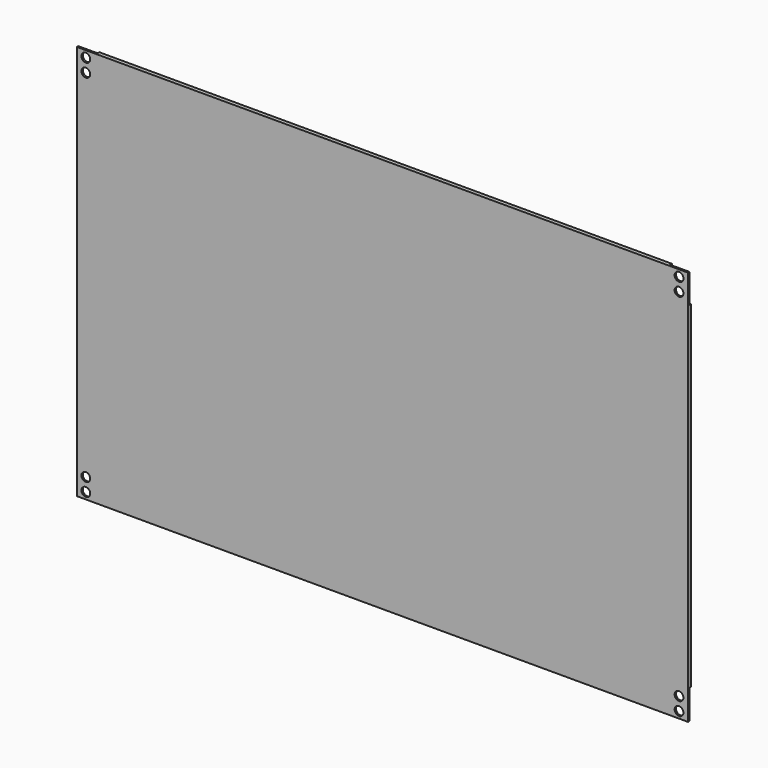
from build123d import *

# Parameters (mm, degrees)
F0_W     = 44
F0_H     = 67
F0_R     = 10
F1_DEPTH = 9
F2_DEPTH = 5


# Not quite as in the source:
# - a feature names something its author has since deleted; it is built from what else it names


with BuildPart() as f1:
    # F0 (on Front) → F1 (new body)
    with BuildSketch(Plane.XZ):
        Polygon((658.4285732806, 488.9782061457), (-644.5714267194, 488.9782061457), (-644.5714267194, 421.9782061457), (-688.5714267194, 421.9782061457), (-688.5714267194, -344.0217938543), (-644.5714267194, -344.0217938543), (-644.5714267194, -411.0217938543), (658.4285732806, -411.0217938543), (658.4285732806, -344.0217938543), (702.4285732806, -344.0217938543), (702.4285732806, 421.9782061457), (658.4285732806, 421.9782061457), align=None)
        with Locations((680.4285732806, -377.5217938543)):
            Rectangle(F0_W, F0_H)
        with Locations((681.9285732806, -396.0217938543)):
            Circle(F0_R, mode=Mode.SUBTRACT)
        with Locations((681.9285732806, -366.0217938543)):
            Circle(F0_R, mode=Mode.SUBTRACT)
        with Locations((-666.5714267194, 455.4782061457)):
            Rectangle(F0_W, F0_H)
        with Locations((-668.0714267194, 443.9782061457)):
            Circle(F0_R, mode=Mode.SUBTRACT)
        with Locations((-668.0714267194, 473.9782061457)):
            Circle(F0_R, mode=Mode.SUBTRACT)
        with Locations((680.4285732806, 455.4782061457)):
            Rectangle(F0_W, F0_H)
        with Locations((681.9285732806, 443.9782061457)):
            Circle(F0_R, mode=Mode.SUBTRACT)
        with Locations((681.9285732806, 473.9782061457)):
            Circle(F0_R, mode=Mode.SUBTRACT)
        with Locations((-666.5714267194, -377.5217938543)):
            Rectangle(F0_W, F0_H)
        with Locations((-668.0714267194, -396.0217938543)):
            Circle(F0_R, mode=Mode.SUBTRACT)
        with Locations((-668.0714267194, -366.0217938543)):
            Circle(F0_R, mode=Mode.SUBTRACT)
    extrude(amount=F1_DEPTH)

    # F0 (on Front) → F2 (cut)
    with BuildSketch(Plane.XZ):
        with Locations((680.4285732806, -377.5217938543)):
            Rectangle(F0_W, F0_H)
        with Locations((681.9285732806, -396.0217938543)):
            Circle(F0_R, mode=Mode.SUBTRACT)
        with Locations((681.9285732806, -366.0217938543)):
            Circle(F0_R, mode=Mode.SUBTRACT)
        with Locations((-666.5714267194, 455.4782061457)):
            Rectangle(F0_W, F0_H)
        with Locations((-668.0714267194, 443.9782061457)):
            Circle(F0_R, mode=Mode.SUBTRACT)
        with Locations((-668.0714267194, 473.9782061457)):
            Circle(F0_R, mode=Mode.SUBTRACT)
        with Locations((680.4285732806, 455.4782061457)):
            Rectangle(F0_W, F0_H)
        with Locations((681.9285732806, 443.9782061457)):
            Circle(F0_R, mode=Mode.SUBTRACT)
        with Locations((681.9285732806, 473.9782061457)):
            Circle(F0_R, mode=Mode.SUBTRACT)
        with Locations((-666.5714267194, -377.5217938543)):
            Rectangle(F0_W, F0_H)
        with Locations((-668.0714267194, -396.0217938543)):
            Circle(F0_R, mode=Mode.SUBTRACT)
        with Locations((-668.0714267194, -366.0217938543)):
            Circle(F0_R, mode=Mode.SUBTRACT)
    extrude(amount=F2_DEPTH, mode=Mode.SUBTRACT)


solid = f1.part
